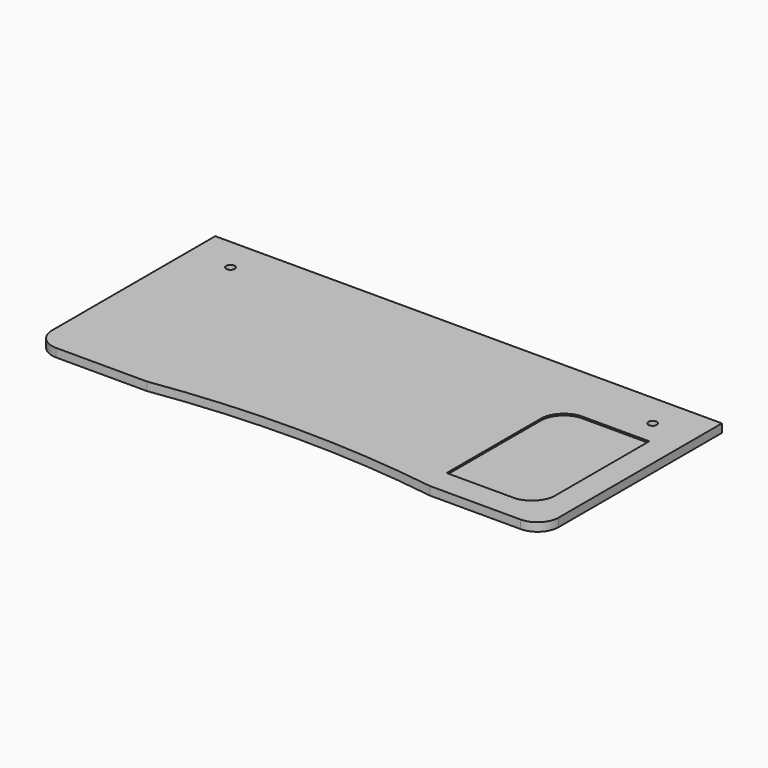
from build123d import *

# Parameters (mm, degrees)
F0_R     = 15
F1_DEPTH = 30
F2_DEPTH = 24
F3_W     = 406
F3_H     = 725
F3_R     = 15
F4_DEPTH = 4


# Not quite as in the source:
# - a feature names something its author has since deleted; it is built from what else it names


with BuildPart() as f1:
    # F0 (on Top) → F1 (new body)
    with BuildSketch(Plane.XY):
        with BuildLine():
            ThreePointArc((4355.1985619355, -294.5215593797), (4377.1655533465, -347.5545679687), (4430.1985619355, -369.5215593797))
            Line((4430.1985619355, -369.5215593797), (4753.0624461818, -369.5215593797))
            ThreePointArc((4753.0624461818, -369.5215593797), (5255.1985619355, -332.6549530029), (5757.3346776893, -369.5215593797))
            Line((5757.3346776893, -369.5215593797), (6080.1985619355, -369.5215593797))
            ThreePointArc((6080.1985619355, -369.5215593797), (6133.2315705245, -347.5545679687), (6155.1985619355, -294.5215593797))
            Line((6155.1985619355, -294.5215593797), (6155.1985619355, 430.4784406203))
            Line((6155.1985619355, 430.4784406203), (4355.1985619355, 430.4784406203))
            Line((4355.1985619355, 430.4784406203), (4355.1985619355, -294.5215593797))
        make_face()
        with BuildLine():
            Line((6065.1985619355, 163.3609871071), (6065.1985619355, -195.1546647585))
            Line((6065.1985619355, -195.1546647585), (6065.1985619355, -204.4389326959))
            Line((6065.1985619355, -204.4389326959), (6065.1159855294, -205.7217836249))
            ThreePointArc((6065.1159855294, -205.7217836249), (6040.8429178387, -255.0832383215), (5991.4814631421, -279.3563060122))
            Line((5991.4814631421, -279.3563060122), (5990.1985619355, -279.5026946765))
            Line((5990.1985619355, -279.5026946765), (5968.0089636665, -279.5215593797))
            Line((5968.0089636665, -279.5215593797), (5745.1985619355, -279.5215593797))
            Line((5745.1985619355, -279.5215593797), (5745.1985619355, 102.1975441552))
            Line((5745.1985619355, 102.1975441552), (5745.2811886192, 146.843918233))
            ThreePointArc((5745.2811886192, 146.843918233), (5769.55425631, 196.2053729296), (5818.9157110066, 220.4784406203))
            Line((5818.9157110066, 220.4784406203), (6065.1985619355, 220.4784406203))
            Line((6065.1985619355, 220.4784406203), (6065.1985619355, 163.3609871071))
        make_face(mode=Mode.SUBTRACT)
        with Locations((4505.1985619355, 310.4784406203)):
            Circle(F0_R, mode=Mode.SUBTRACT)
        with Locations((6005.1985619355, 310.4784406203)):
            Circle(F0_R, mode=Mode.SUBTRACT)
    extrude(amount=F1_DEPTH)

    # F0 (on Top) → F2 (join)
    with BuildSketch(Plane.XY):
        with BuildLine():
            Line((6065.1985619355, -204.4389326959), (6065.1985619355, -195.1546647585))
            Line((6065.1985619355, -195.1546647585), (6065.1985619355, 163.3609871071))
            Line((6065.1985619355, 163.3609871071), (6065.1985619355, 220.4784406203))
            Line((6065.1985619355, 220.4784406203), (5818.9157110066, 220.4784406203))
            ThreePointArc((5818.9157110066, 220.4784406203), (5769.55425631, 196.2053729296), (5745.2811886192, 146.843918233))
            Line((5745.2811886192, 146.843918233), (5745.1985619355, 102.1975441552))
            Line((5745.1985619355, 102.1975441552), (5745.1985619355, -279.5215593797))
            Line((5745.1985619355, -279.5215593797), (5968.0089636665, -279.5215593797))
            Line((5968.0089636665, -279.5215593797), (5990.1985619355, -279.5026946765))
            Line((5990.1985619355, -279.5026946765), (5991.4814631421, -279.3563060122))
            ThreePointArc((5991.4814631421, -279.3563060122), (6040.8429178387, -255.0832383215), (6065.1159855294, -205.7217836249))
            Line((6065.1159855294, -205.7217836249), (6065.1985619355, -204.4389326959))
        make_face()
    extrude(amount=F2_DEPTH)

    # F3 (on face) + F0 (on Top) → F4 (cut)
    with BuildSketch(Plane.XY):
        with Locations((5902.1985619355, 57.9784406203)):
            Rectangle(F3_W, F3_H)
        with BuildLine():
            Line((6065.1985619355, 220.4784406203), (6065.1985619355, 163.3609871071))
            Line((6065.1985619355, 163.3609871071), (6065.1985619355, -195.1546647585))
            Line((6065.1985619355, -195.1546647585), (6065.1985619355, -204.4389326959))
            Line((6065.1985619355, -204.4389326959), (6065.1159855294, -205.7217836249))
            ThreePointArc((6065.1159855294, -205.7217836249), (6040.8429178387, -255.0832383215), (5991.4814631421, -279.3563060122))
            Line((5991.4814631421, -279.3563060122), (5990.1985619355, -279.5026946765))
            Line((5990.1985619355, -279.5026946765), (5968.0089636665, -279.5215593797))
            Line((5968.0089636665, -279.5215593797), (5745.1985619355, -279.5215593797))
            Line((5745.1985619355, -279.5215593797), (5745.1985619355, 102.1975441552))
            Line((5745.1985619355, 102.1975441552), (5745.2811886192, 146.843918233))
            ThreePointArc((5745.2811886192, 146.843918233), (5769.55425631, 196.2053729296), (5818.9157110066, 220.4784406203))
            Line((5818.9157110066, 220.4784406203), (6065.1985619355, 220.4784406203))
        make_face(mode=Mode.SUBTRACT)
        with Locations((6005.1985619355, 310.4784406203)):
            Circle(F3_R, mode=Mode.SUBTRACT)
    with BuildSketch(Plane.XY):
        with BuildLine():
            Line((6065.1985619355, -204.4389326959), (6065.1985619355, -195.1546647585))
            Line((6065.1985619355, -195.1546647585), (6065.1985619355, 163.3609871071))
            Line((6065.1985619355, 163.3609871071), (6065.1985619355, 220.4784406203))
            Line((6065.1985619355, 220.4784406203), (5818.9157110066, 220.4784406203))
            ThreePointArc((5818.9157110066, 220.4784406203), (5769.55425631, 196.2053729296), (5745.2811886192, 146.843918233))
            Line((5745.2811886192, 146.843918233), (5745.1985619355, 102.1975441552))
            Line((5745.1985619355, 102.1975441552), (5745.1985619355, -279.5215593797))
            Line((5745.1985619355, -279.5215593797), (5968.0089636665, -279.5215593797))
            Line((5968.0089636665, -279.5215593797), (5990.1985619355, -279.5026946765))
            Line((5990.1985619355, -279.5026946765), (5991.4814631421, -279.3563060122))
            ThreePointArc((5991.4814631421, -279.3563060122), (6040.8429178387, -255.0832383215), (6065.1159855294, -205.7217836249))
            Line((6065.1159855294, -205.7217836249), (6065.1985619355, -204.4389326959))
        make_face()
    extrude(amount=F4_DEPTH, mode=Mode.SUBTRACT)


solid = f1.part
